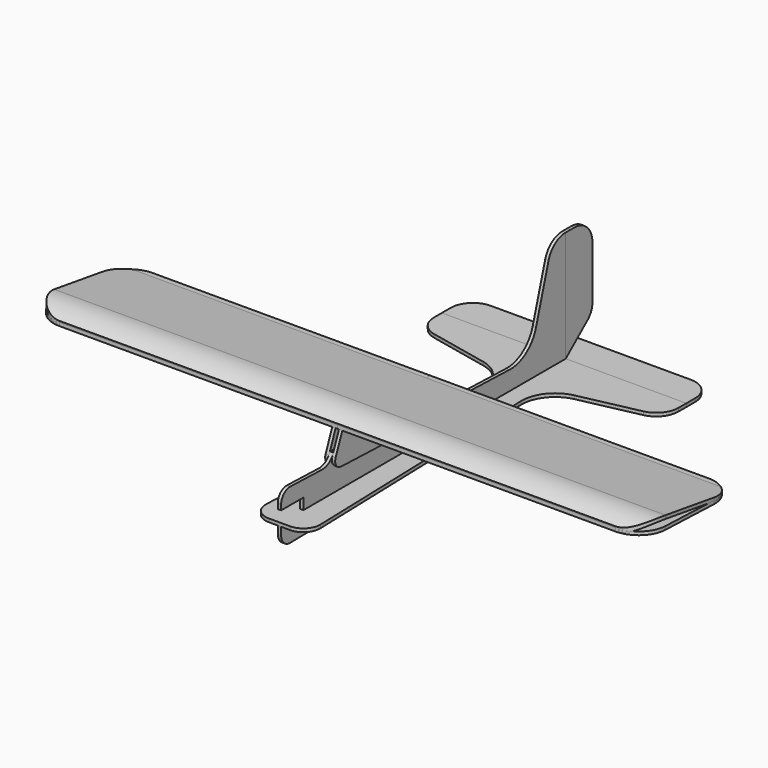
from build123d import *

# Parameters (mm, degrees)
F6_DEPTH  = 1.5
F7_DEPTH  = 1.5
F8_DEPTH  = 1.5
F9_DEPTH  = 3
F10_DEPTH = 3
F11_DEPTH = 400
F12_DEPTH = 25
F13_START = 1.5
F13_DEPTH = 3
F15_DEPTH = 3
F16_DEPTH = 3


with BuildPart() as f6:
    # F1 (on Right) → F6 (new body, symmetric)
    with BuildSketch(Plane.YZ):
        with BuildLine():
            Line((25, 0), (320, 0))
            Line((320, 0), (320, 15))
            Line((320, 15), (320, 100))
            Line((320, 100), (319.901906, 100))
            ThreePointArc((319.901906, 100), (307.952308, 96.037678), (300.737526, 85.720711))
            Line((300.737526, 85.720711), (286.604631, 38.375515))
            ThreePointArc((286.604631, 38.375515), (275.404526, 22.623032), (256.921018, 16.971218))
            Line((256.921018, 16.971218), (183.402692, 19.268666))
            ThreePointArc((183.402692, 19.268666), (176.376671, 21.596288), (171.75982, 27.381397))
            Line((171.75982, 27.381397), (171.497773, 28.02828))
            Line((171.497773, 28.02828), (58.557854, 31.972228))
            Line((58.557854, 31.972228), (58.41841, 31.6316))
            ThreePointArc((58.41841, 31.6316), (53.462774, 25.650759), (45.981439, 23.56308))
            Line((45.981439, 23.56308), (10.312348, 24.677739))
            ThreePointArc((10.312348, 24.677739), (3.04024, 21.863269), (0, 14.682618))
            Line((0, 14.682618), (0, 10))
            Line((0, 10), (25, 10))
            Line((25, 10), (25, 0))
        make_face()
    extrude(amount=F6_DEPTH, both=True)


with BuildPart() as f7:
    # F1 (on Right) → F7 (new body, symmetric)
    with BuildSketch(Plane.YZ):
        with BuildLine():
            Line((0, -3), (0, -9.842529))
            ThreePointArc((0, -9.842529), (2.984386, -16.968619), (10.156231, -19.841309))
            Line((10.156231, -19.841309), (310.156231, -15.153809))
            ThreePointArc((310.156231, -15.153809), (317.12609, -12.170644), (320, -5.155029))
            Line((320, -5.155029), (320, -3))
            Line((320, -3), (0, -3))
        make_face()
    extrude(amount=F7_DEPTH, both=True)


with BuildPart() as f8:
    # F1 (on Right) → F8 (new body, symmetric)
    with BuildSketch(Plane.YZ):
        with BuildLine():
            Line((320, 15), (320, 0))
            Line((320, 0), (344.641814, 20.676937))
            ThreePointArc((344.641814, 20.676937), (348.594617, 25.82833), (350, 32.167604))
            Line((350, 32.167604), (350, 80))
            ThreePointArc((350, 80), (344.142136, 94.142136), (330, 100))
            Line((330, 100), (320, 100))
            Line((320, 100), (320, 15))
        make_face()
    extrude(amount=F8_DEPTH, both=True)


with BuildPart() as f9:
    # F3 (on Top) → F9 (new body)
    with BuildSketch(Plane.XY):
        with BuildLine():
            Line((0, 320), (0, 0))
            Line((0, 0), (9.523928, 0))
            ThreePointArc((9.523928, 0), (20.294903, 4.56036), (24.516609, 15.468521))
            Line((24.516609, 15.468521), (17.188737, 249.960421))
            ThreePointArc((17.188737, 249.960421), (23.557651, 269.397824), (40.904952, 280.235115))
            Line((40.904952, 280.235115), (94.179432, 291.619311))
            ThreePointArc((94.179432, 291.619311), (105.549737, 298.599761), (110, 311.177745))
            Line((110, 311.177745), (110, 320))
            Line((110, 320), (3, 320))
            Line((3, 320), (0, 320))
        make_face()
        with BuildLine():
            Line((-9.523928, 0), (0, 0))
            Line((0, 0), (0, 320))
            Line((0, 320), (-3, 320))
            Line((-3, 320), (-110, 320))
            Line((-110, 320), (-110, 311.177745))
            ThreePointArc((-110, 311.177745), (-105.549737, 298.599761), (-94.179432, 291.619311))
            Line((-94.179432, 291.619311), (-40.904952, 280.235115))
            ThreePointArc((-40.904952, 280.235115), (-23.557651, 269.397824), (-17.188737, 249.960421))
            Line((-17.188737, 249.960421), (-24.516609, 15.468521))
            ThreePointArc((-24.516609, 15.468521), (-20.294903, 4.56036), (-9.523928, 0))
        make_face()
    extrude(amount=-F9_DEPTH)


with BuildPart() as f10:
    # F3 (on Top) → F10 (new body)
    with BuildSketch(Plane.XY):
        with BuildLine():
            Line((-3, 320), (0, 320))
            Line((0, 320), (3, 320))
            Line((3, 320), (27.142136, 344.142136))
            ThreePointArc((27.142136, 344.142136), (33.630603, 348.477591), (41.284271, 350))
            Line((41.284271, 350), (-41.284271, 350))
            ThreePointArc((-41.284271, 350), (-33.630603, 348.477591), (-27.142136, 344.142136))
            Line((-27.142136, 344.142136), (-3, 320))
        make_face()
        with BuildLine():
            Line((27.142136, 344.142136), (3, 320))
            Line((3, 320), (110, 320))
            Line((110, 320), (110, 330))
            ThreePointArc((110, 330), (104.142136, 344.142136), (90, 350))
            Line((90, 350), (41.284271, 350))
            ThreePointArc((41.284271, 350), (33.630603, 348.477591), (27.142136, 344.142136))
        make_face()
        with BuildLine():
            Line((-110, 320), (-3, 320))
            Line((-3, 320), (-27.142136, 344.142136))
            ThreePointArc((-27.142136, 344.142136), (-33.630603, 348.477591), (-41.284271, 350))
            Line((-41.284271, 350), (-90, 350))
            ThreePointArc((-90, 350), (-104.142136, 344.142136), (-110, 330))
            Line((-110, 330), (-110, 320))
        make_face()
    extrude(amount=-F10_DEPTH)


with BuildPart() as f11:
    # F2 (on Right) → F11 (new body, symmetric)
    with BuildSketch(Plane.YZ):
        with BuildLine():
            Line((89.895891, 55.438452), (164.939083, 44.218885))
            Line((164.939083, 44.218885), (165.382677, 47.185908))
            Line((165.382677, 47.185908), (90.339485, 58.405475))
            ThreePointArc((90.339485, 58.405475), (75.674959, 57.284155), (62.954005, 49.902896))
            Line((62.954005, 49.902896), (65, 47.708835))
            ThreePointArc((65, 47.708835), (76.564504, 54.41907), (89.895891, 55.438452))
        make_face()
    extrude(amount=F11_DEPTH, both=True)

    # F5 (on line) → F12 (intersect)
    with BuildSketch(Plane(origin=(0, 1.743168, 49.917812), x_dir=(1, 0, 0), z_dir=(0, 0.034899, 0.999391))):
        with BuildLine():
            Line((0, 103.295389), (0, 63.295389))
            Line((0, 63.295389), (250, 63.295389))
            ThreePointArc((250, 63.295389), (267.67767, 70.61772), (275, 88.295389))
            Line((275, 88.295389), (275, 103.295389))
            Line((275, 103.295389), (0, 103.295389))
        make_face()
        with BuildLine():
            Line((0, 168.295389), (0, 103.295389))
            Line((0, 103.295389), (275, 103.295389))
            Line((275, 103.295389), (275, 143.295389))
            ThreePointArc((275, 143.295389), (267.67767, 160.973059), (250, 168.295389))
            Line((250, 168.295389), (0, 168.295389))
        make_face()
        with BuildLine():
            Line((-250, 63.295389), (0, 63.295389))
            Line((0, 63.295389), (0, 103.295389))
            Line((0, 103.295389), (-275, 103.295389))
            Line((-275, 103.295389), (-275, 88.295389))
            ThreePointArc((-275, 88.295389), (-267.67767, 70.61772), (-250, 63.295389))
        make_face()
        with BuildLine():
            Line((-275, 103.295389), (0, 103.295389))
            Line((0, 103.295389), (0, 168.295389))
            Line((0, 168.295389), (-250, 168.295389))
            ThreePointArc((-250, 168.295389), (-267.67767, 160.973059), (-275, 143.295389))
            Line((-275, 143.295389), (-275, 103.295389))
        make_face()
    extrude(amount=F12_DEPTH, mode=Mode.INTERSECT)


with BuildPart() as f13:
    # F2 (on Right) → F13 (new body)
    with BuildSketch(Plane.YZ.offset(F13_START)):
        with BuildLine():
            Line((172.380518, 25.849159), (164.939083, 44.218885))
            Line((164.939083, 44.218885), (89.895891, 55.438452))
            ThreePointArc((89.895891, 55.438452), (76.564504, 54.41907), (65, 47.708835))
            Line((65, 47.708835), (57.517657, 29.431279))
            ThreePointArc((57.517657, 29.431279), (58.11642, 22.980286), (63.751548, 19.783546))
            Line((63.751548, 19.783546), (165.648339, 16.225232))
            ThreePointArc((165.648339, 16.225232), (171.628539, 19.20856), (172.380518, 25.849159))
        make_face()
    extrude(amount=F13_DEPTH)


with BuildPart() as f14_1:
    # F14: instance of F13
    add(f13.part.mirror(Plane.YZ))


with BuildPart() as f15:
    # F5 (on line) → F15 (new body)
    with BuildSketch(Plane(origin=(0, 1.743168, 49.917812), x_dir=(1, 0, 0), z_dir=(0, 0.034899, 0.999391))):
        with BuildLine():
            Line((-250, 63.295389), (0, 63.295389))
            Line((0, 63.295389), (0, 103.295389))
            Line((0, 103.295389), (-275, 103.295389))
            Line((-275, 103.295389), (-275, 88.295389))
            ThreePointArc((-275, 88.295389), (-267.67767, 70.61772), (-250, 63.295389))
        make_face()
        with BuildLine():
            Line((-275, 103.295389), (0, 103.295389))
            Line((0, 103.295389), (0, 168.295389))
            Line((0, 168.295389), (-250, 168.295389))
            ThreePointArc((-250, 168.295389), (-267.67767, 160.973059), (-275, 143.295389))
            Line((-275, 143.295389), (-275, 103.295389))
        make_face()
    extrude(amount=F15_DEPTH)


with BuildPart() as f16:
    # F5 (on line) → F16 (new body)
    with BuildSketch(Plane(origin=(0, 1.743168, 49.917812), x_dir=(1, 0, 0), z_dir=(0, 0.034899, 0.999391))):
        with BuildLine():
            Line((0, 103.295389), (0, 63.295389))
            Line((0, 63.295389), (250, 63.295389))
            ThreePointArc((250, 63.295389), (267.67767, 70.61772), (275, 88.295389))
            Line((275, 88.295389), (275, 103.295389))
            Line((275, 103.295389), (0, 103.295389))
        make_face()
        with BuildLine():
            Line((0, 168.295389), (0, 103.295389))
            Line((0, 103.295389), (275, 103.295389))
            Line((275, 103.295389), (275, 143.295389))
            ThreePointArc((275, 143.295389), (267.67767, 160.973059), (250, 168.295389))
            Line((250, 168.295389), (0, 168.295389))
        make_face()
    extrude(amount=F16_DEPTH)


solid = Compound([f6.part, f7.part, f8.part, f9.part, f10.part, f11.part, f13.part, f14_1.part, f15.part, f16.part])
